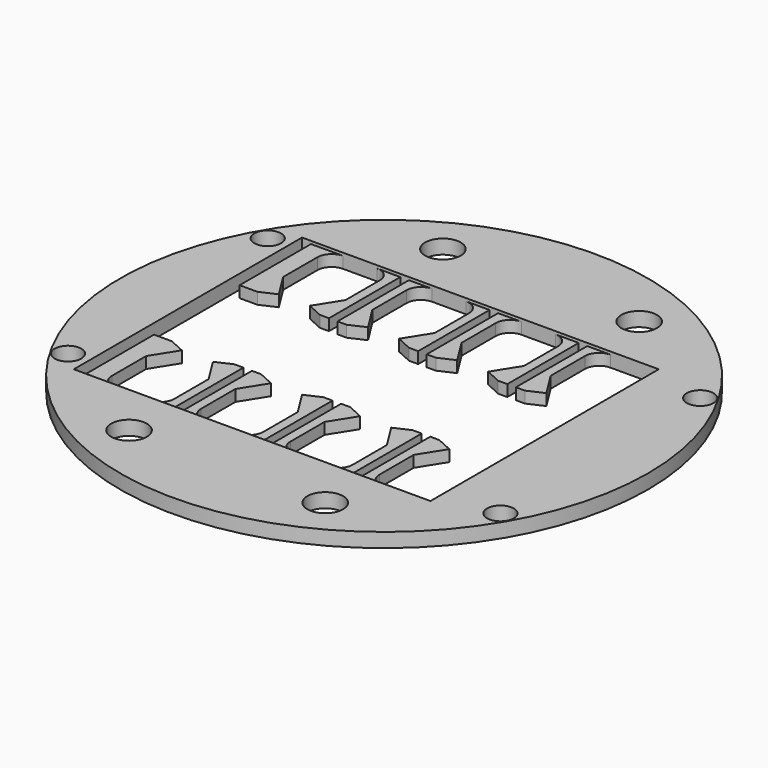
from build123d import *

# Parameters (mm, degrees)
F0_R     = 52.3875
F1_DEPTH = 2.54
F2_R     = 2.54
F3_W     = 63.5
F3_H     = 50.8
F4_DEPTH = 0.508
F5_R     = 52.3875
F5_R_2   = 46.99
F5_R_3   = 2.38125
F5_R_4   = 3.175
F6_DEPTH = 25.4
F7_W     = 1.524
F7_H     = 15.875
F8_DEPTH = 25.4


# Not quite as in the source:
# - a feature names something its author has since deleted; it is built from what else it names


with BuildPart() as f1:
    # F0 (on Top) → F1 (new body)
    with BuildSketch(Plane.XY):
        Circle(F0_R)
        Polygon((-34.925, 25.4), (-33.3375, 25.4), (-30.1625, 25.4), (-19.05, 25.4), (-19.05, 15.24), (-21.844, 10.795), (-19.05, 9.525), (-17.4625, 9.525), (-14.2875, 9.525), (-11.4935, 10.795), (-14.2875, 15.24), (-14.2875, 25.4), (-3.175, 25.4), (-3.175, 15.24), (-5.969, 10.795), (-3.175, 9.525), (-1.5875, 9.525), (1.5875, 9.525), (4.3815, 10.795), (1.5875, 15.24), (1.5875, 25.4), (12.7, 25.4), (12.7, 15.24), (9.906, 10.795), (12.7, 9.525), (14.2875, 9.525), (17.4625, 9.525), (20.2565, 10.795), (17.4625, 15.24), (17.4625, 25.4), (28.575, 25.4), (28.575, -25.4), (17.4625, -25.4), (17.4625, -15.24), (20.2565, -10.795), (17.4625, -9.525), (14.2875, -9.525), (12.7, -9.525), (9.906, -10.795), (12.7, -15.24), (12.7, -25.4), (1.5875, -25.4), (1.5875, -15.24), (4.3815, -10.795), (1.5875, -9.525), (-1.5875, -9.525), (-3.175, -9.525), (-5.969, -10.795), (-3.175, -15.24), (-3.175, -25.4), (-14.2875, -25.4), (-14.2875, -15.24), (-11.4935, -10.795), (-14.2875, -9.525), (-17.4625, -9.525), (-19.05, -9.525), (-21.844, -10.795), (-19.05, -15.24), (-19.05, -25.4), (-30.1625, -25.4), (-33.3375, -25.4), (-34.925, -25.4), align=None, mode=Mode.SUBTRACT)
        Polygon((-33.3375, 9.525), (-30.1625, 9.525), (-27.3685, 10.795), (-30.1625, 15.24), (-30.1625, 25.4), (-33.3375, 25.4), align=None)
        Polygon((-33.3375, -9.525), (-33.3375, -25.4), (-30.1625, -25.4), (-30.1625, -15.24), (-27.3685, -10.795), (-30.1625, -9.525), align=None)
    extrude(amount=F1_DEPTH)

    # F2
    f2_edges = [f1.edges().sort_by_distance(p)[0] for p in [
        (-30.1625, 25.4, 1.27),
        (-14.2875, 25.4, 1.27),
        (1.5875, 25.4, 1.27),
        (17.4625, 25.4, 1.27),
        (17.4625, -25.4, 1.27),
        (1.5875, -25.4, 1.27),
        (-14.2875, -25.4, 1.27),
        (-30.1625, -25.4, 1.27),
        (-19.05, -25.4, 1.27),
        (-3.175, -25.4, 1.27),
        (12.7, -25.4, 1.27),
        (12.7, 25.4, 1.27),
        (-3.175, 25.4, 1.27),
        (-19.05, 25.4, 1.27),
    ]]
    fillet(f2_edges, radius=F2_R)

    # F3 (on face) → F4 (cut)
    with BuildSketch(Plane.XY.offset(2.54)):
        with Locations((-3.175, 0)):
            Rectangle(F3_W, F3_H)
    extrude(amount=-F4_DEPTH, mode=Mode.SUBTRACT)

    # F5 (on face) → F6 (cut)
    with BuildSketch(Plane.XY.offset(2.54)):
        Circle(F5_R)
        Circle(F5_R_2, mode=Mode.SUBTRACT)
        with Locations((-38.4948291982, 22.225)):
            Circle(F5_R_3)
        with Locations((-38.4948291982, -22.225)):
            Circle(F5_R_3)
        with Locations((38.4948291982, -22.225)):
            Circle(F5_R_3)
        with Locations((38.4948291982, 22.225)):
            Circle(F5_R_3)
        with Locations((17.4625, -34.925)):
            Circle(F5_R_4)
        with Locations((17.4625, 34.925)):
            Circle(F5_R_4)
        with Locations((-17.4625, 34.925)):
            Circle(F5_R_4)
        with Locations((-17.4625, -34.925)):
            Circle(F5_R_4)
    extrude(amount=-F6_DEPTH, mode=Mode.SUBTRACT)

    # F7 (on face) → F8 (cut)
    with BuildSketch(Plane.XY.offset(2.54)):
        with Locations((-16.66875, 17.4625)):
            Rectangle(F7_W, F7_H)
        with Locations((-0.79375, 17.4625)):
            Rectangle(F7_W, F7_H)
        with Locations((15.08125, 17.4625)):
            Rectangle(F7_W, F7_H)
        with Locations((-16.66875, -17.4625)):
            Rectangle(F7_W, F7_H)
        with Locations((-0.79375, -17.4625)):
            Rectangle(F7_W, F7_H)
        with Locations((15.08125, -17.4625)):
            Rectangle(F7_W, F7_H)
    extrude(amount=-F8_DEPTH, mode=Mode.SUBTRACT)


solid = f1.part
